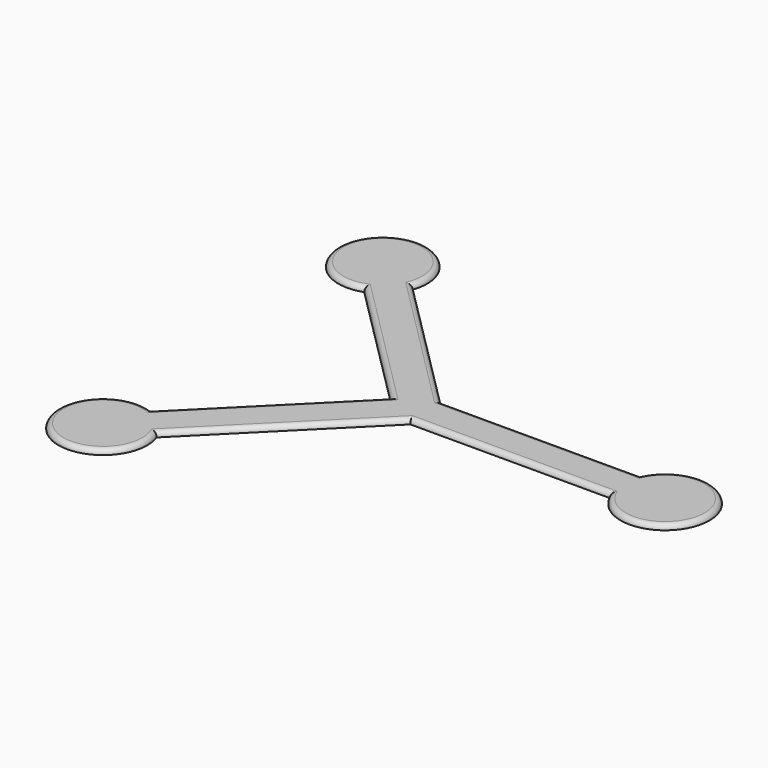
from build123d import *

# Parameters (mm, degrees)
F1_DEPTH = 4
F2_R     = 3.99999


# Not quite as in the source:
# - a fillet or chamfer is up to 0.001 mm smaller than in the source, because OpenCascade refuses the exact size


with BuildPart() as f1:
    # F0 (on Top) → F1 (new body)
    with BuildSketch(Plane.XY):
        with BuildLine():
            Line((6.2132034356, -15), (163.3772233983, -15))
            ThreePointArc((163.3772233983, -15), (230, 0), (163.3772233983, 15))
            Line((163.3772233983, 15), (6.2132034356, 15))
            Line((6.2132034356, 15), (-104.9185408386, 126.1317442742))
            ThreePointArc((-104.9185408386, 126.1317442742), (-162.6345596729, 162.6345596729), (-126.1317442742, 104.9185408386))
            Line((-126.1317442742, 104.9185408386), (-21.2132034356, 0))
            Line((-21.2132034356, 0), (-126.1317442742, -104.9185408386))
            ThreePointArc((-126.1317442742, -104.9185408386), (-162.6345596729, -162.6345596729), (-104.9185408386, -126.1317442742))
            Line((-104.9185408386, -126.1317442742), (6.2132034356, -15))
        make_face()
    extrude(amount=F1_DEPTH)

    # F2 (radius 4 in the source; OpenCascade refuses exactly that, so slightly less here)
    f2_edges = [f1.edges().sort_by_distance(p)[0] for p in [
        (-49.352669, -70.565872, 4),
        (84.795213, -15, 4),
        (230, 0, 4),
        (84.795213, 15, 4),
        (-49.352669, 70.565872, 4),
        (-162.63456, 162.63456, 4),
        (-73.672474, 52.45927, 4),
        (-73.672474, -52.45927, 4),
        (-162.63456, -162.63456, 4),
    ]]
    fillet(f2_edges, radius=F2_R)


solid = f1.part
